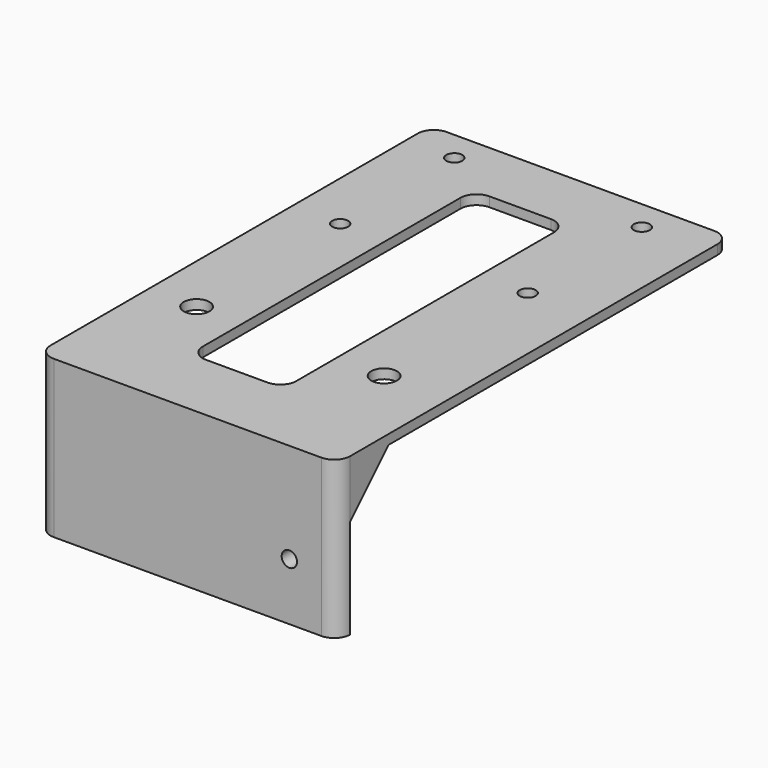
from build123d import *

# Parameters (mm, degrees)
F0_W     = 93.5
F0_H     = 153.21
F0_R     = 4
F0_R_2   = 2.5
F0_W_2   = 29.1728788614
F0_H_2   = 110.4717357084
F1_DEPTH = 3
F2_W     = 93.5
F2_H     = 5
F3_DEPTH = 46
F4_R     = 2.4
F5_DEPTH = 5
F6_W     = 3
F6_H     = 15
F7_DEPTH = 15
F9_DEPTH = 93.501
F10_R    = 4.99999


# Not quite as in the source:
# - a fillet or chamfer is up to 0.001 mm smaller than in the source, because OpenCascade refuses the exact size


with BuildPart() as f1:
    # F0 (on Top) → F1 (new body)
    with BuildSketch(Plane.XY):
        with Locations((-46.75, 76.605)):
            Rectangle(F0_W, F0_H)
        with Locations((-78.5, 43.21)):
            Circle(F0_R, mode=Mode.SUBTRACT)
        with Locations((-20, 43.21)):
            Circle(F0_R, mode=Mode.SUBTRACT)
        with Locations((-78.5, 99.21)):
            Circle(F0_R_2, mode=Mode.SUBTRACT)
        with Locations((-49.5864394307, 77.9741321458)):
            Rectangle(F0_W_2, F0_H_2, mode=Mode.SUBTRACT)
        with Locations((-78.5, 143.71)):
            Circle(F0_R_2, mode=Mode.SUBTRACT)
        with Locations((-20, 99.21)):
            Circle(F0_R_2, mode=Mode.SUBTRACT)
        with Locations((-20, 143.71)):
            Circle(F0_R_2, mode=Mode.SUBTRACT)
    extrude(amount=-F1_DEPTH)

    # F2 (on face) → F3 (join)
    with BuildSketch(Plane(origin=(0, 0, -3), x_dir=(1, 0, 0), z_dir=(0, 0, -1))):
        with Locations((-46.75, -2.5)):
            Rectangle(F2_W, F2_H)
    extrude(amount=F3_DEPTH)

    # F4 (on face) → F5 (cut, through all)
    with BuildSketch(Plane.XZ):
        with Locations((-15, -31.12)):
            Circle(F4_R)
    extrude(amount=-F5_DEPTH, mode=Mode.SUBTRACT)

    # F6 (on face) → F7 (join)
    with BuildSketch(Plane(origin=(0, 5, 0), x_dir=(-1, 0, 0), z_dir=(0, 1, 0))):
        with Locations((1.5, -10.5)):
            Rectangle(F6_W, F6_H)
        with Locations((92, -10.5)):
            Rectangle(F6_W, F6_H)
    extrude(amount=F7_DEPTH)

    # F8 (on face) → F9 (cut, through all)
    with BuildSketch(Plane(origin=(-93.5, 0, 0), x_dir=(0, -1, 0), z_dir=(-1, 0, 0))):
        Polygon((-5, -18), (-20, -3), (-20, -18), align=None)
    extrude(amount=-F9_DEPTH, mode=Mode.SUBTRACT)

    # F10 (radius 5 in the source; OpenCascade refuses exactly that, so slightly less here)
    f10_edges = [f1.edges().sort_by_distance(p)[0] for p in [
        (0, 153.21, -1.5),
        (-93.5, 153.21, -1.5),
        (0, 0, -24.5),
        (-93.5, 0, -24.5),
        (-64.172879, 133.21, -1.5),
        (-64.172879, 22.738264, -1.5),
        (-35, 22.738264, -1.5),
        (-35, 133.21, -1.5),
    ]]
    fillet(f10_edges, radius=F10_R)


solid = f1.part
